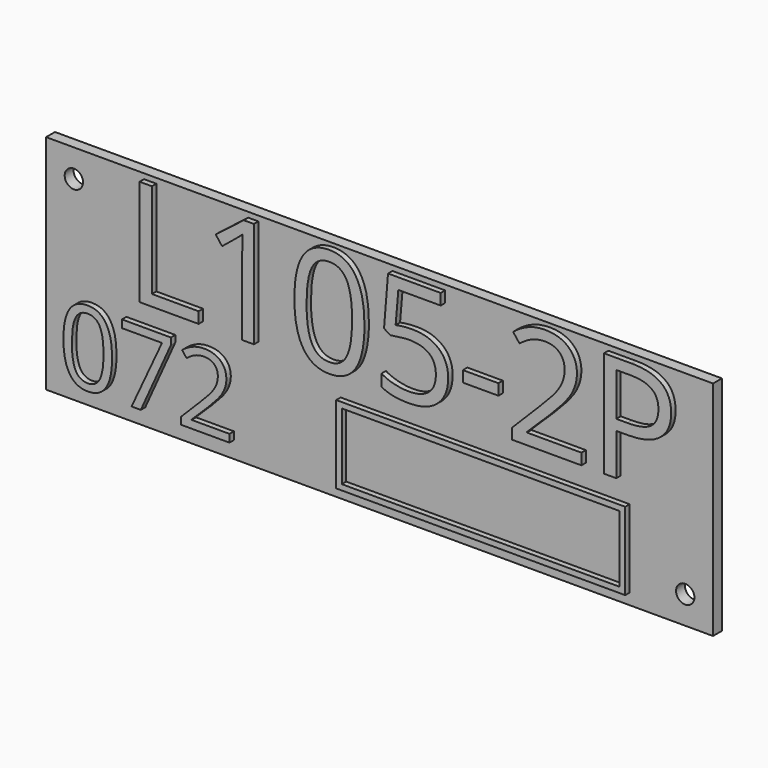
from build123d import *

# Parameters (mm, degrees)
F0_W         = 120
F0_H         = 40
F1_DEPTH     = 2
F3_D         = 3.3
F4_TEXT_SIZE = 26.7145301999
F5_DEPTH     = 1
F6_TEXT_SIZE = 18.5356140827
F7_DEPTH     = 1
F8_W         = 52
F8_H         = 14
F8_W_2       = 49.99999962
F8_H_2       = 11.99999962
F9_DEPTH     = 1


# Not quite as in the source:
# - Text() gives the source's letters only with a copy of the font that has no kerning and outlines rounded to 1/6400 em; it was checked with that copy


with BuildPart() as f1:
    # F0 (on Front) → F1 (new body)
    with BuildSketch(Plane.XZ):
        Rectangle(F0_W, F0_H)
    extrude(amount=F1_DEPTH)

    # F3 (through all)
    with Locations(Plane.XZ.offset(2)):
        with Locations((-55, 15), (55, -15)):
            Hole(F3_D / 2)

    # F4 (on face) → F5 (join)
    with BuildSketch(Plane.XZ.offset(2)):
        with Locations((-45, 0)):
            Text('L105-2P', F4_TEXT_SIZE, font='Open Sans', text_align=(TextAlign.LEFT, TextAlign.BOTTOM))
    extrude(amount=F5_DEPTH)

    # F6 (on face) → F7 (join)
    with BuildSketch(Plane.XZ.offset(2)):
        with Locations((-57, -17)):
            Text('072', F6_TEXT_SIZE, font='Open Sans', text_align=(TextAlign.LEFT, TextAlign.BOTTOM))
    extrude(amount=F7_DEPTH)

    # F8 (on face) → F9 (join)
    with BuildSketch(Plane.XZ.offset(2)):
        with Locations((19, -11)):
            Rectangle(F8_W, F8_H)
        with Locations((19, -11)):
            Rectangle(F8_W_2, F8_H_2, mode=Mode.SUBTRACT)
    extrude(amount=F9_DEPTH)


solid = f1.part
